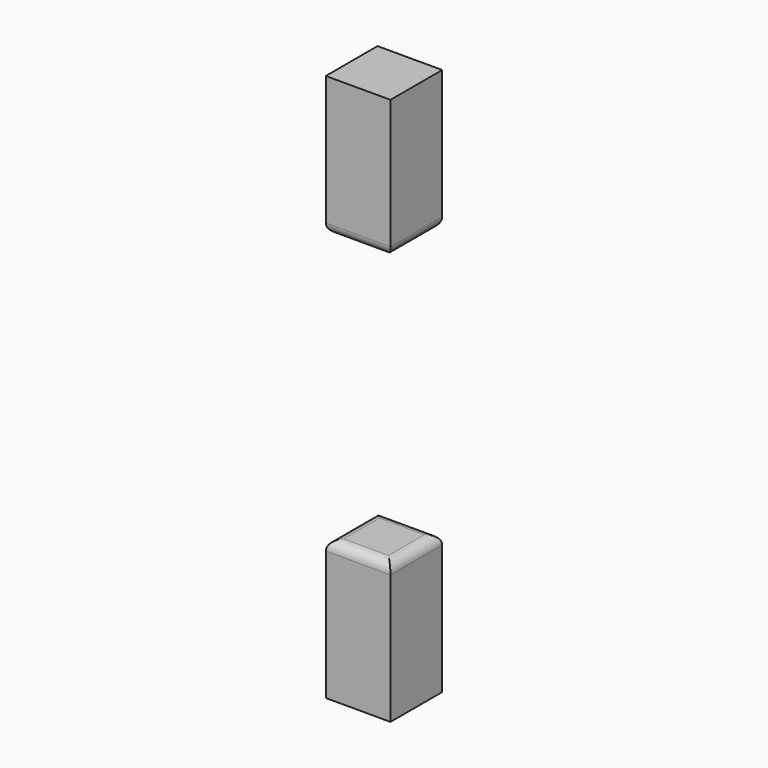
from build123d import *

# Parameters (mm, degrees)
F2_W     = 82.55
F2_H     = 82.55
F3_DEPTH = 177.8
F4_W     = 82.55
F4_H     = 82.55
F5_DEPTH = 177.8
F6_R     = 12.7
F7_R     = 12.7


# Not quite as in the source:
# - the program builds the solid bodies; features that only make, move or delete a surface that nothing else refers to are left out


with BuildPart() as f3:
    # F2 (on face) → F3 (new body)
    with BuildSketch(Plane(origin=(0, 0, -115.5637845452), x_dir=(1, 0, 0), z_dir=(0, 0, -1))):
        Rectangle(F2_W, F2_H)
    extrude(amount=F3_DEPTH)

    # F7
    f7_edges = [f3.edges().sort_by_distance(p)[0] for p in [
        (0, 41.275, -115.563785),
        (41.275, 0, -115.563785),
        (0, -41.275, -115.563785),
        (-41.275, 0, -115.563785),
    ]]
    fillet(f7_edges, radius=F7_R)


with BuildPart() as f5:
    # F4 (on face) → F5 (new body)
    with BuildSketch(Plane.XY.offset(227.7861535549)):
        Rectangle(F4_W, F4_H)
    extrude(amount=F5_DEPTH)

    # F6
    f6_edges = [f5.edges().sort_by_distance(p)[0] for p in [
        (0, -41.275, 227.786154),
        (41.275, 0, 227.786154),
        (0, 41.275, 227.786154),
        (-41.275, 0, 227.786154),
    ]]
    fillet(f6_edges, radius=F6_R)


solid = Compound([f3.part, f5.part])
